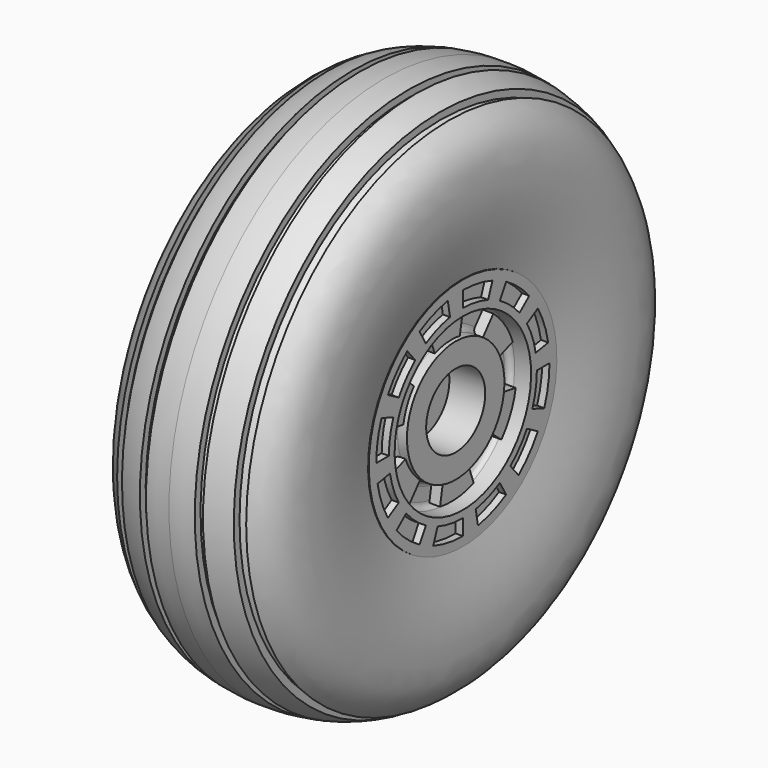
from build123d import *

# Parameters (mm, degrees)
F2_W            = 0.2
F2_H            = 0.22
F3_ANGLE        = 20
F3_COPIES_COUNT = 12
F5_DEPTH        = 0.15


# Not quite as in the source:
# - a pattern or mirror of a feature is missing from the dataset's text; its kind, count and spacing are read off the source's solid


with BuildPart() as f1:
    # F0 (on Front) → F1 (revolve)
    with BuildSketch(Plane.XZ):
        with BuildLine():
            Line((1, 0.85), (0.87, 0.85))
            ThreePointArc((0.87, 0.85), (0.8134314575, 0.8734314575), (0.79, 0.93))
            Line((0.79, 0.93), (0.79, 1.11))
            ThreePointArc((0.79, 1.11), (0.8134314575, 1.1665685425), (0.87, 1.19))
            Line((0.87, 1.19), (1.1, 1.19))
            Line((1.1, 1.19), (1.1, 1.59))
            Line((1.1, 1.59), (1.1, 1.64))
            Line((1.1, 1.64), (1.0898001841, 1.64))
            add(Edge.make_bspline(
                [(1.0898001841, 1.64), (1.25, 2.278713374), (1.2631809244, 2.7012833679), (1.2262611325, 3.2585699441), (0.9876698715, 3.4728439225), (0.9, 3.5283316002)],
                knots=[0, 0, 0, 0, 0.3702653747, 0.6271589839, 0.7357428034, 0.7357428034, 0.7357428034, 0.7357428034], degree=3))
            Line((0.9, 3.5283316002), (0.9, 3.4283316002))
            Line((0.9, 3.4283316002), (0.78, 3.4941282527))
            Line((0.78, 3.4941282527), (0.78, 3.5941282527))
            add(Edge.make_bspline(
                [(0.78, 3.5941282527), (0.6808228027, 3.641181915), (0.5666603708, 3.6793418914), (0.44, 3.7061262113)],
                knots=[0.7816518304, 0.7816518304, 0.7816518304, 0.7816518304, 0.8878685464, 0.8878685464, 0.8878685464, 0.8878685464], degree=3))
            Line((0.44, 3.7061262113), (0.44, 3.6061262113))
            Line((0.44, 3.6061262113), (0.34, 3.6244667725))
            Line((0.34, 3.6244667725), (0.34, 3.7244667725))
            add(Edge.make_bspline(
                [(0.34, 3.7244667725), (0.2338131535, 3.7410670641), (0.120057055, 3.75), (0, 3.75)],
                knots=[0.9151424409, 0.9151424409, 0.9151424409, 0.9151424409, 1, 1, 1, 1], degree=3))
            Line((0, 3.75), (0, 0.515))
            Line((0, 0.515), (0, 0))
            Line((0, 0), (0.5, 0))
            Line((0.5, 0), (0.5, 0.515))
            Line((0.5, 0.515), (1, 0.515))
            Line((1, 0.515), (1, 0.85))
        make_face()
    revolve(axis=Axis((1.042, 0, 0), (1, 0, 0)))

    # F2 (on Front) → F3 (revolve, cut)
    with BuildSketch(Plane.XZ):
        with Locations((1.1, 1.4)):
            Rectangle(F2_W, F2_H)
    f3 = revolve(axis=Axis((1.36, 0, 0), (-1, 0, 0)), revolution_arc=F3_ANGLE, mode=Mode.SUBTRACT)

    # F3_copies: F3 ×12 about axis
    f3_copies_axis = Axis((0, 0, 0), (1, 0, 0))
    for i in range(1, F3_COPIES_COUNT):
        add(f3.rotate(f3_copies_axis, i * 360 / F3_COPIES_COUNT), mode=Mode.SUBTRACT)

    # F4 (on face) → F5 (join)
    with BuildSketch(Plane.YZ.offset(0.79)):
        with BuildLine():
            Line((-0.3895609432, 1.0703098951), (-0.2696546218, 0.7408699845))
            ThreePointArc((-0.2696546218, 0.7408699845), (-0.0687151015, 0.7854172037), (0.1369072395, 0.7764395384))
            Line((0.1369072395, 0.7764395384), (0.1977852744, 1.1216960307))
            ThreePointArc((0.1977852744, 1.1216960307), (-0.099270391, 1.1346657611), (-0.3895609432, 1.0703098951))
        make_face()
        with BuildLine():
            Line((-1.1216960307, 0.1977852744), (-0.7764395384, 0.1369072395))
            ThreePointArc((-0.7764395384, 0.1369072395), (-0.7145488017, 0.3331995784), (-0.603962745, 0.5067849166))
            Line((-0.603962745, 0.5067849166), (-0.8725246207, 0.7321350874))
            ThreePointArc((-0.8725246207, 0.7321350874), (-1.0322845694, 0.4813622001), (-1.1216960307, 0.1977852744))
        make_face()
        with BuildLine():
            Line((-0.7321350874, -0.8725246207), (-0.5067849166, -0.603962745))
            ThreePointArc((-0.5067849166, -0.603962745), (-0.6458337002, -0.4522176253), (-0.7408699845, -0.2696546218))
            Line((-0.7408699845, -0.2696546218), (-1.0703098951, -0.3895609432))
            ThreePointArc((-1.0703098951, -0.3895609432), (-0.9330141784, -0.653303561), (-0.7321350874, -0.8725246207))
        make_face()
        with BuildLine():
            Line((0.3895609432, -1.0703098951), (0.2696546218, -0.7408699845))
            ThreePointArc((0.2696546218, -0.7408699845), (0.0687151015, -0.7854172037), (-0.1369072395, -0.7764395384))
            Line((-0.1369072395, -0.7764395384), (-0.1977852744, -1.1216960307))
            ThreePointArc((-0.1977852744, -1.1216960307), (0.099270391, -1.1346657611), (0.3895609432, -1.0703098951))
        make_face()
        with BuildLine():
            Line((1.1216960307, -0.1977852744), (0.7764395384, -0.1369072395))
            ThreePointArc((0.7764395384, -0.1369072395), (0.7145488017, -0.3331995784), (0.603962745, -0.5067849166))
            Line((0.603962745, -0.5067849166), (0.8725246207, -0.7321350874))
            ThreePointArc((0.8725246207, -0.7321350874), (1.0322845694, -0.4813622001), (1.1216960307, -0.1977852744))
        make_face()
        with BuildLine():
            Line((0.7321350874, 0.8725246207), (0.5067849166, 0.603962745))
            ThreePointArc((0.5067849166, 0.603962745), (0.6458337002, 0.4522176253), (0.7408699845, 0.2696546218))
            Line((0.7408699845, 0.2696546218), (1.0703098951, 0.3895609432))
            ThreePointArc((1.0703098951, 0.3895609432), (0.9330141784, 0.653303561), (0.7321350874, 0.8725246207))
        make_face()
    extrude(amount=F5_DEPTH)

    # F6: F1 across face


with BuildPart() as f1_1:
    add(f1.part)
    add(f1.part.mirror(Plane(origin=(0, 0, 0), x_dir=(0, -1, 0), z_dir=(-1, 0, 0))))


solid = f1_1.part
